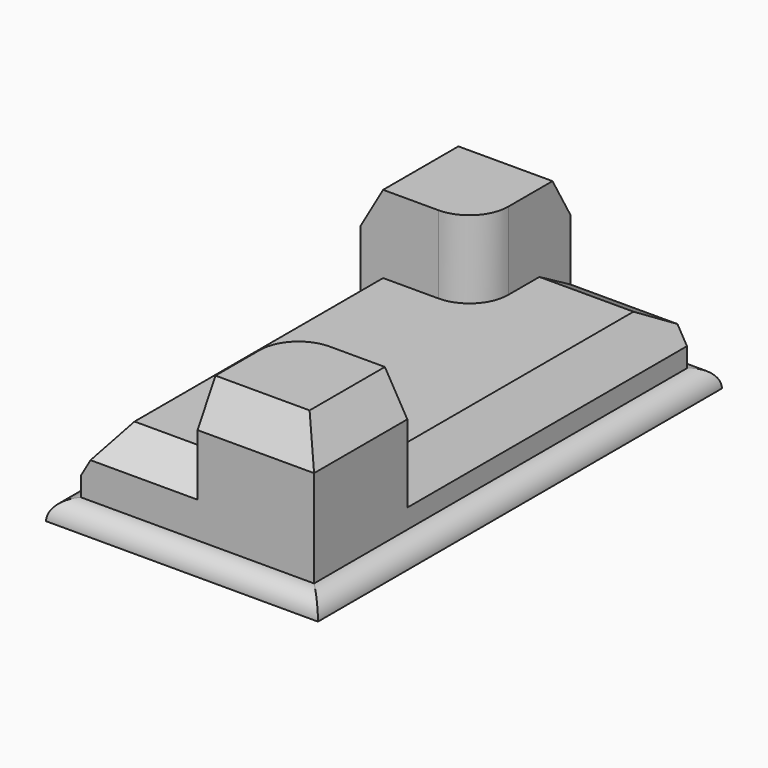
from build123d import *

# Parameters (mm, degrees)
F0_W        = 88.9
F0_H        = 165.1
F1_DEPTH    = 6.35
F2_DEPTH    = 25.4
F3_DEPTH    = 50.8
F4_C1_SIZE2 = 7.3323484187
F4_C1_SIZE  = 12.7
F4_C2_SIZE2 = 7.3323484187
F4_C2_SIZE  = 12.7
F4_C3_SIZE2 = 12.7
F4_C3_SIZE  = 7.3323484187
F4_C4_SIZE2 = 7.3323484187
F4_C4_SIZE  = 12.7
F5_C1_SIZE2 = 12.7
F5_C1_SIZE  = 7.3323484187
F5_C2_SIZE2 = 7.3323484187
F5_C2_SIZE  = 12.7
F5_C3_SIZE2 = 7.3323484187
F5_C3_SIZE  = 12.7
F5_C4_SIZE2 = 7.3323484187
F5_C4_SIZE  = 12.7
F6_R        = 6.34999


# Not quite as in the source:
# - a fillet or chamfer is up to 0.001 mm smaller than in the source, because OpenCascade refuses the exact size


with BuildPart() as f1:
    # F0 (on Top) → F1 (new body)
    with BuildSketch(Plane.XY):
        Rectangle(F0_W, F0_H)
        Polygon((0, 76.2), (38.1, 76.2), (38.1, -38.1), (38.1, -76.2), (0, -76.2), (-38.1, -76.2), (-38.1, 38.1), (-38.1, 76.2), align=None, mode=Mode.SUBTRACT)
    extrude(amount=F1_DEPTH)

    # F0 (on Top) → F2 (join)
    with BuildSketch(Plane.XY):
        with BuildLine():
            Line((38.1, -38.1), (38.1, 76.2))
            Line((38.1, 76.2), (0, 76.2))
            Line((0, 76.2), (0, 50.8))
            ThreePointArc((0, 50.8), (-3.7197438789, 41.8197438789), (-12.7, 38.1))
            Line((-12.7, 38.1), (-38.1, 38.1))
            Line((-38.1, 38.1), (-38.1, -76.2))
            Line((-38.1, -76.2), (0, -76.2))
            Line((0, -76.2), (0, -50.8))
            ThreePointArc((0, -50.8), (3.7197438789, -41.8197438789), (12.7, -38.1))
            Line((12.7, -38.1), (38.1, -38.1))
        make_face()
    extrude(amount=F2_DEPTH)

    # F0 (on Top) → F3 (join)
    with BuildSketch(Plane.XY):
        with BuildLine():
            Line((0, 50.8), (0, 76.2))
            Line((0, 76.2), (-38.1, 76.2))
            Line((-38.1, 76.2), (-38.1, 38.1))
            Line((-38.1, 38.1), (-12.7, 38.1))
            ThreePointArc((-12.7, 38.1), (-3.7197438789, 41.8197438789), (0, 50.8))
        make_face()
        with BuildLine():
            Line((38.1, -76.2), (38.1, -38.1))
            Line((38.1, -38.1), (12.7, -38.1))
            ThreePointArc((12.7, -38.1), (3.7197438789, -41.8197438789), (0, -50.8))
            Line((0, -50.8), (0, -76.2))
            Line((0, -76.2), (38.1, -76.2))
        make_face()
    extrude(amount=F3_DEPTH)

    # F4: chamfer of 12.7 x 7.3323484187 on 4 edges, made by hand

    # F4_c1
    f4_c1_edges = [f1.edges().sort_by_distance(p)[0] for p in [
        (-38.1, 57.15, 50.8),
    ]]
    f4_c1_side = f1.faces().sort_by_distance((-38.1, 57.15, 50.6533530316))[0]
    chamfer(f4_c1_edges, length=F4_C1_SIZE, length2=F4_C1_SIZE2, reference=f4_c1_side)

    # F4_c2
    f4_c2_edges = [f1.edges().sort_by_distance(p)[0] for p in [
        (-38.1, -19.05, 25.4),
    ]]
    f4_c2_side = f1.faces().sort_by_distance((-38.1, -19.05, 25.2533530316))[0]
    chamfer(f4_c2_edges, length=F4_C2_SIZE, length2=F4_C2_SIZE2, reference=f4_c2_side)

    # F4_c3
    f4_c3_edges = [f1.edges().sort_by_distance(p)[0] for p in [
        (-15.3838257906, -76.2, 25.4),
    ]]
    f4_c3_side = f1.faces().sort_by_distance((-15.3838257906, -76.2, 25.2533530316))[0]
    chamfer(f4_c3_edges, length=F4_C3_SIZE, length2=F4_C3_SIZE2, reference=f4_c3_side)

    # F4_c4
    f4_c4_edges = [f1.edges().sort_by_distance(p)[0] for p in [
        (-15.3838257906, 76.2, 50.8),
    ]]
    f4_c4_side = f1.faces().sort_by_distance((-15.3838257906, 76.2, 50.6533530316))[0]
    chamfer(f4_c4_edges, length=F4_C4_SIZE, length2=F4_C4_SIZE2, reference=f4_c4_side)

    # F5: chamfer of 12.7 x 7.3323484187 on 4 edges, made by hand

    # F5_c1
    f5_c1_edges = [f1.edges().sort_by_distance(p)[0] for p in [
        (19.05, 76.2, 25.4),
    ]]
    f5_c1_side = f1.faces().sort_by_distance((19.05, 76.2, 25.2533530316))[0]
    chamfer(f5_c1_edges, length=F5_C1_SIZE, length2=F5_C1_SIZE2, reference=f5_c1_side)

    # F5_c2
    f5_c2_edges = [f1.edges().sort_by_distance(p)[0] for p in [
        (38.1, 12.7, 25.4),
    ]]
    f5_c2_side = f1.faces().sort_by_distance((38.1, 12.7, 25.2533530316))[0]
    chamfer(f5_c2_edges, length=F5_C2_SIZE, length2=F5_C2_SIZE2, reference=f5_c2_side)

    # F5_c3
    f5_c3_edges = [f1.edges().sort_by_distance(p)[0] for p in [
        (38.1, -57.15, 50.8),
    ]]
    f5_c3_side = f1.faces().sort_by_distance((38.1, -57.15, 50.6533530316))[0]
    chamfer(f5_c3_edges, length=F5_C3_SIZE, length2=F5_C3_SIZE2, reference=f5_c3_side)

    # F5_c4
    f5_c4_edges = [f1.edges().sort_by_distance(p)[0] for p in [
        (15.3838257906, -76.2, 50.8),
    ]]
    f5_c4_side = f1.faces().sort_by_distance((15.3838257906, -76.2, 50.6533530316))[0]
    chamfer(f5_c4_edges, length=F5_C4_SIZE, length2=F5_C4_SIZE2, reference=f5_c4_side)

    # F6 (radius 6.35 in the source; OpenCascade refuses exactly that, so slightly less here)
    f6_edges = [f1.edges().sort_by_distance(p)[0] for p in [
        (-44.45, 0, 6.35),
        (0, -82.55, 6.35),
        (0, 82.55, 6.35),
        (44.45, 0, 6.35),
    ]]
    fillet(f6_edges, radius=F6_R)


solid = f1.part
